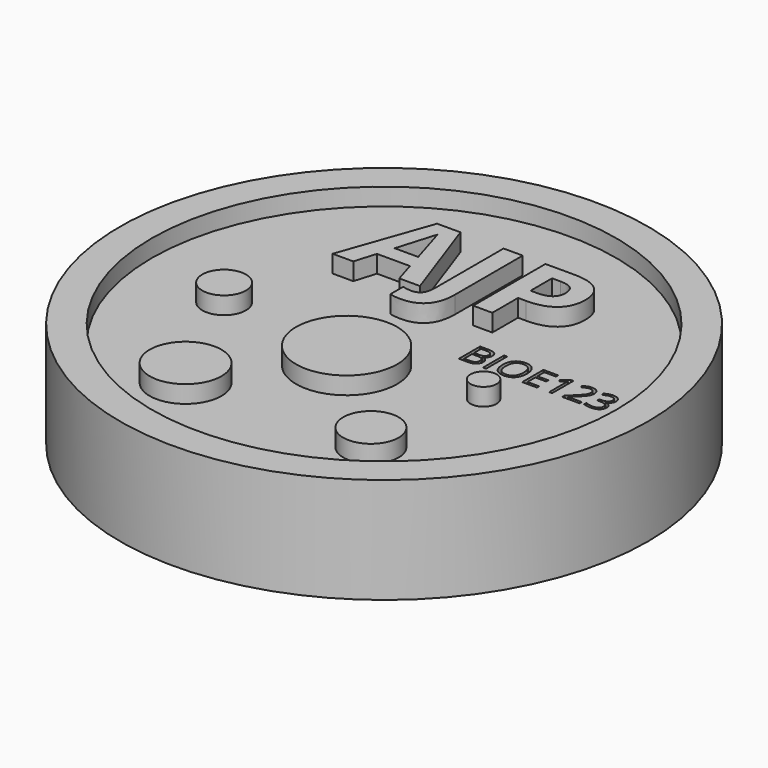
from build123d import *

# Parameters (mm, degrees)
F0_R         = 25
F0_R_2       = 22
F1_DEPTH     = 10
F0_R_3       = 3.4027575679
F0_R_4       = 2.0681032813
F0_R_5       = 2.6267836514
F0_R_6       = 4.7876110968
F0_R_7       = 1.2393390337
F2_DEPTH     = 2
F3_DEPTH     = 10
F4_TEXT_SIZE = 11.9838966389
F5_DEPTH     = 10
F6_DEPTH     = 6.35
F7_TEXT_SIZE = 3.5149660665
F8_DEPTH     = 3.175


# Not quite as in the source:
# - Text() gives the source's letters only with a copy of the font that has no kerning and outlines rounded to 1/6400 em; it was checked with that copy


with BuildPart() as f1:
    # F0 (on Top) → F1 (new body)
    with BuildSketch(Plane.XY):
        Circle(F0_R)
        Circle(F0_R_2, mode=Mode.SUBTRACT)
    extrude(amount=F1_DEPTH)

    # F0 (on Top) → F2 (join)
    with BuildSketch(Plane.XY):
        Circle(F0_R_2)
        with Locations((-7.5708734803, -14.0381408855)):
            Circle(F0_R_3, mode=Mode.SUBTRACT)
        with Locations((-13.389791362, -2.2030537948)):
            Circle(F0_R_4, mode=Mode.SUBTRACT)
        with Locations((9.5900027081, -13.5450111702)):
            Circle(F0_R_5, mode=Mode.SUBTRACT)
        with Locations((0, -4.4362442568)):
            Circle(F0_R_6, mode=Mode.SUBTRACT)
        with Locations((11.2666403875, -2.3016794585)):
            Circle(F0_R_7, mode=Mode.SUBTRACT)
    extrude(amount=F2_DEPTH)

    # F0 (on Top) → F3 (join)
    with BuildSketch(Plane.XY):
        with Locations((-13.389791362, -2.2030537948)):
            Circle(F0_R_4)
        with Locations((-7.5708734803, -14.0381408855)):
            Circle(F0_R_3)
        with Locations((0, -4.4362442568)):
            Circle(F0_R_6)
        with Locations((11.2666403875, -2.3016794585)):
            Circle(F0_R_7)
        with Locations((9.5900027081, -13.5450111702)):
            Circle(F0_R_5)
    extrude(amount=F3_DEPTH)

    # F4 (on Top) → F5 (join)
    with BuildSketch(Plane.XY):
        with Locations((-10, 6.4062640513)):
            Text('AJP', F4_TEXT_SIZE, font='Open Sans', font_style=FontStyle.BOLD, text_align=(TextAlign.LEFT, TextAlign.BOTTOM))
    extrude(amount=F5_DEPTH)


with BuildPart() as f6:
    # F6 (new): a face of the model
    f6_faces = [f1.part.faces().sort_by_distance(p)[0] for p in [
        (-21.3777460297, 0, 2),
    ]]
    extrude(f6_faces, amount=F6_DEPTH)

    # F7 (on face) → F8 (cut)
    with BuildSketch(Plane.XY.offset(8.35)):
        with Locations((5.4715560274, 1.5874468391)):
            Text('BIOE123', F7_TEXT_SIZE, font='Open Sans', text_align=(TextAlign.LEFT, TextAlign.BOTTOM))
    extrude(amount=-F8_DEPTH, mode=Mode.SUBTRACT)


solid = Compound([f1.part, f6.part])
